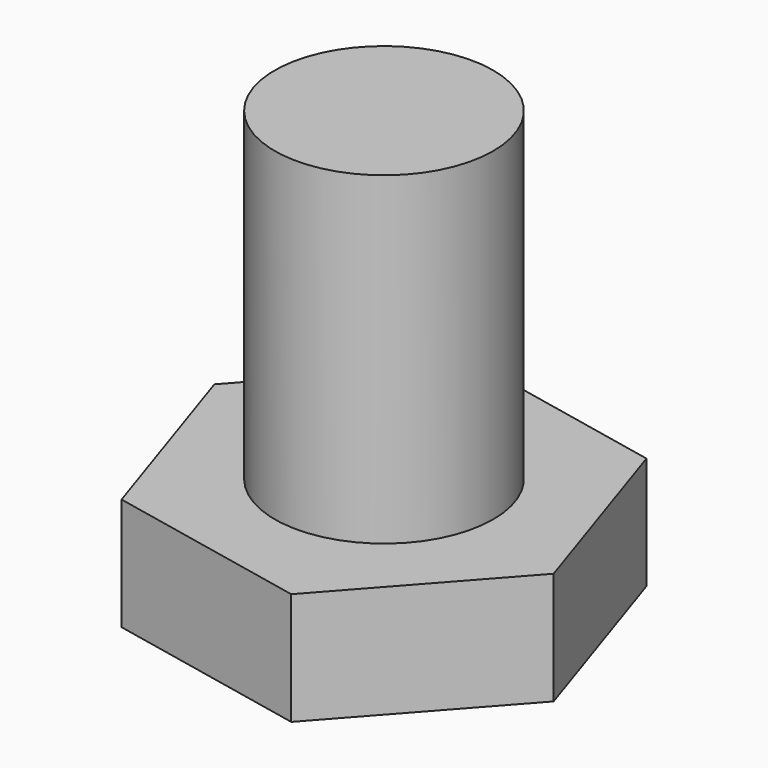
from build123d import *

# Parameters (mm, degrees)
F1_DEPTH = 81.026
F2_R     = 78.74
F3_DEPTH = 233.68
F4_R     = 124.3645263244
F5_DEPTH = 2.286
F7_R     = 5.08


# Not quite as in the source:
# - a fillet or chamfer that OpenCascade refuses, or shapes differently, is made with other operations: its cross-section is extruded or revolved along the edge and cut away or added


with BuildPart() as f1:
    # F0 (on Top) → F1 (new body)
    with BuildSketch(Plane.XY):
        Polygon((46.9164714903, -142.236754682), (146.6388786516, -30.4875211745), (99.7224071613, 111.7492335075), (-46.9164714903, 142.236754682), (-146.6388786516, 30.4875211745), (-99.7224071613, -111.7492335075), align=None)
    extrude(amount=F1_DEPTH)

    # F2 (on face) → F3 (join)
    with BuildSketch(Plane.XY.offset(81.026)):
        Circle(F2_R)
    extrude(amount=F3_DEPTH)

    # F4 (on face) → F5 (join)
    with BuildSketch(Plane(origin=(0, 0, 0), x_dir=(1, 0, 0), z_dir=(0, 0, -1))):
        Circle(F4_R)
    extrude(amount=F5_DEPTH)

    # F6: fillet of radius 10.6614809392 on 1 edges, made by hand

    # F6_s1 → F6_t2 (revolve, cut)
    with BuildSketch(Plane.XZ):
        with BuildLine():
            ThreePointArc((124.3645263244, 0), (121.2585269877, -1.6983020197), (117.767671403, -2.286))
            Line((117.767671403, -2.286), (124.3645263244, -2.286))
            Line((124.3645263244, -2.286), (124.3645263244, 0))
        make_face()
    revolve(axis=Axis((0, 0, -2.286), (0, 0, -1)), mode=Mode.SUBTRACT)

    # F7
    f7_edges = [f1.edges().sort_by_distance(p)[0] for p in [
        (-124.364526, 0, 0),
    ]]
    fillet(f7_edges, radius=F7_R)


solid = f1.part
